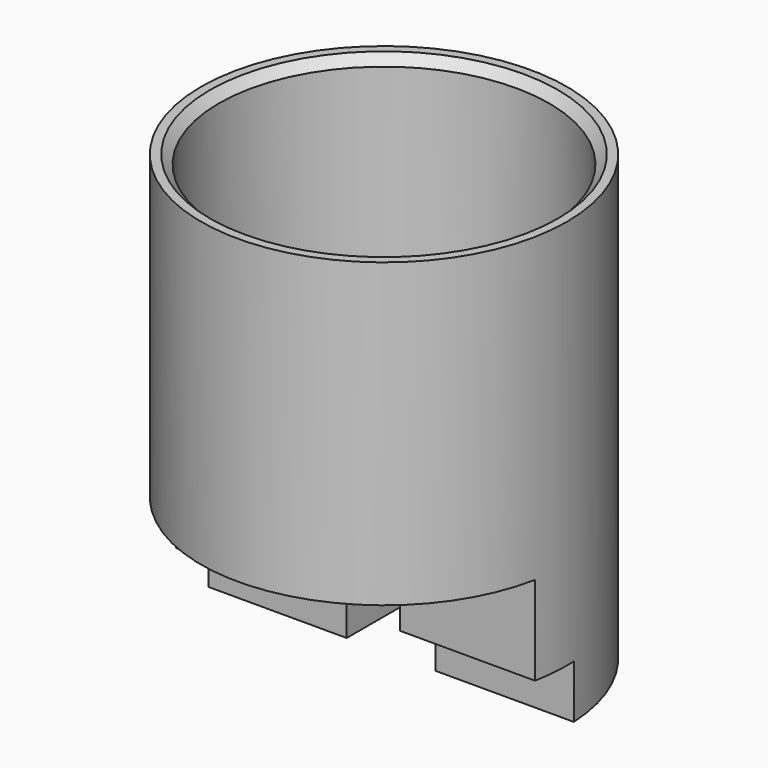
from build123d import *

# Parameters (mm, degrees)
F3_DEPTH  = 18
F4_W      = 8.3
F4_H      = 8
F5_DEPTH  = 10.3
F6_W      = 7.6039596199
F6_H      = 3
F6_W_2    = 0.1960403801
F7_DEPTH  = 2.5
F8_SIZE   = 0.5
F9_R      = 1
F10_DEPTH = 10


# Not quite as in the source:
# - a feature names something its author has since deleted; it is built from what else it names


with BuildPart() as f1:
    # F0 (on Front) → F1 (revolve)
    with BuildSketch(Plane.XZ):
        Polygon((-10.3, 0), (-1.3, 0), (-1.3, 9), (-4.3, 9), (-4.3, 15), (-9.3, 15), (-9.3, 25), (-10.3, 25), align=None)
    revolve(axis=Axis((0, 0, 8.3402672317), (0, 0, 1)))

    # F2 (on Front) → F3 (cut, symmetric)
    with BuildSketch(Plane.XZ):
        with BuildLine():
            Line((-2.5, 5), (-2.5, 0))
            Line((-2.5, 0), (0, 0))
            Line((0, 0), (2.5, 0))
            Line((2.5, 0), (2.5, 5))
            ThreePointArc((2.5, 5), (0, 2.5), (-2.5, 5))
        make_face()
        with BuildLine():
            ThreePointArc((2.5, 5), (0, 7.5), (-2.5, 5))
            ThreePointArc((-2.5, 5), (0, 2.5), (2.5, 5))
        make_face()
    extrude(amount=F3_DEPTH, both=True, mode=Mode.SUBTRACT)

    # F4 (on Right) → F5 (cut, symmetric)
    with BuildSketch(Plane.YZ):
        with Locations((-6.15, 4)):
            Rectangle(F4_W, F4_H)
    extrude(amount=F5_DEPTH, both=True, mode=Mode.SUBTRACT)

    # F6 (on face) → F7 (cut)
    with BuildSketch(Plane.XZ.offset(2)):
        with Locations((6.3019798099, 1.5)):
            Rectangle(F6_W, F6_H)
        with Locations((-6.3019798099, 1.5)):
            Rectangle(F6_W, F6_H)
        with Locations((10.2019798099, 1.5)):
            Rectangle(F6_W_2, F6_H)
        with Locations((-10.2019798099, 1.5)):
            Rectangle(F6_W_2, F6_H)
    extrude(amount=-F7_DEPTH, mode=Mode.SUBTRACT)

    # F8
    f8_edges = [f1.edges().sort_by_distance(p)[0] for p in [
        (9.3, 0, 25),
    ]]
    chamfer(f8_edges, length=F8_SIZE)

    # F9 (on face) → F10 (cut)
    with BuildSketch(Plane(origin=(0, 0, 0), x_dir=(1, 0, 0), z_dir=(0, 0, -1))):
        with Locations((-5, -2.5)):
            Circle(F9_R)
        with Locations((5, -2.5)):
            Circle(F9_R)
    extrude(amount=-F10_DEPTH, mode=Mode.SUBTRACT)


solid = f1.part
